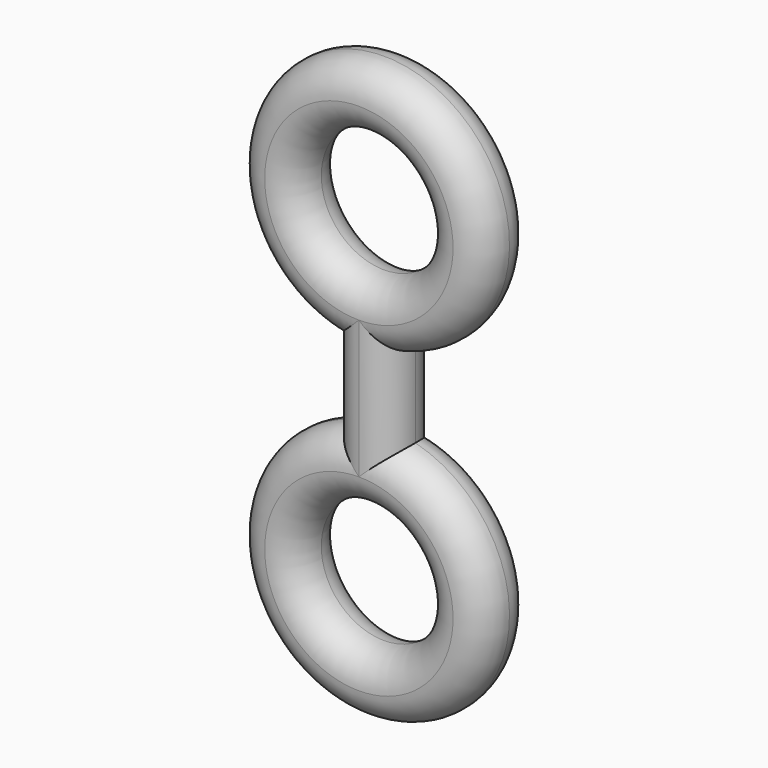
from build123d import *

# Parameters (mm, degrees)
F0_R     = 3.175
F1_DEPTH = 3.175
F2_R     = 1.58749
F3_R     = 1.58749


# Not quite as in the source:
# - a fillet or chamfer is up to 0.001 mm smaller than in the source, because OpenCascade refuses the exact size


with BuildPart() as f1:
    # F0 (on Front) → F1 (new body)
    with BuildSketch(Plane.XZ):
        with BuildLine():
            Line((-1.5875, 2.1066389379), (-1.5875, -2.1066389379))
            ThreePointArc((-1.5875, -2.1066389379), (0, -14.605), (1.5875, -2.1066389379))
            Line((1.5875, -2.1066389379), (1.5875, 2.1066389379))
            ThreePointArc((1.5875, 2.1066389379), (0, 14.605), (-1.5875, 2.1066389379))
        make_face()
        with Locations((0, -8.255)):
            Circle(F0_R, mode=Mode.SUBTRACT)
        with Locations((0, 8.255)):
            Circle(F0_R, mode=Mode.SUBTRACT)
    extrude(amount=F1_DEPTH)

    # F2 (radius 1.5875 in the source; OpenCascade refuses exactly that, so slightly less here)
    f2_edges = [f1.edges().sort_by_distance(p)[0] for p in [
        (-3.175, 0, 8.255),
        (-3.175, 0, -8.255),
        (-3.175, -3.175, 8.255),
        (-3.175, -3.175, -8.255),
    ]]
    fillet(f2_edges, radius=F2_R)

    # F3 (radius 1.5875 in the source; OpenCascade refuses exactly that, so slightly less here)
    f3_edges = [f1.edges().sort_by_distance(p)[0] for p in [
        (0, -3.175, 14.605),
        (-1.5875, -3.175, 0),
        (1.5875, -3.175, 0),
        (0, -3.175, -14.605),
        (0, 0, 14.605),
        (0, 0, -14.605),
        (-1.5875, 0, 0),
        (1.5875, 0, 0),
    ]]
    fillet(f3_edges, radius=F3_R)


solid = f1.part
